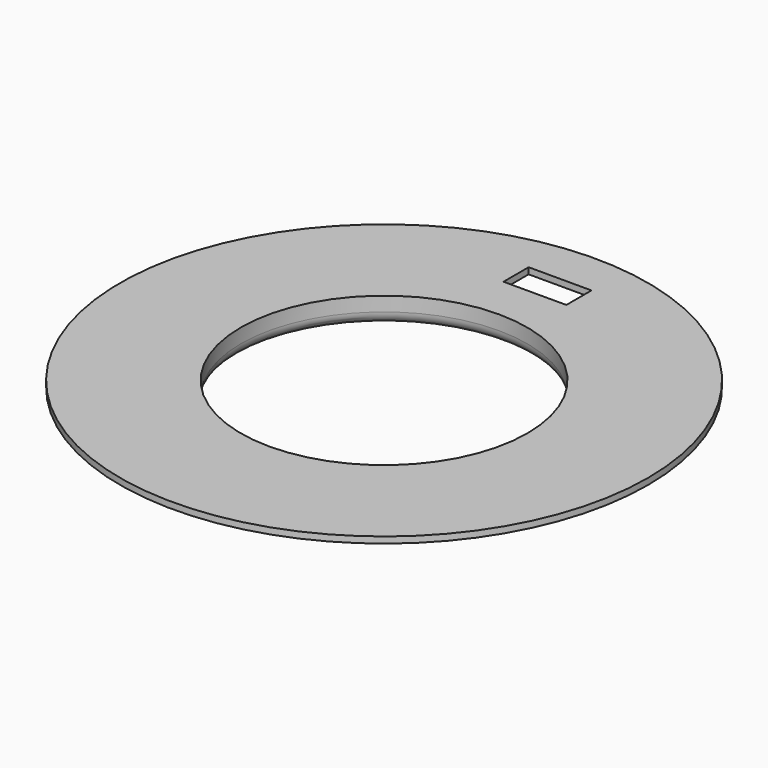
from build123d import *

# Parameters (mm, degrees)
F3_DEPTH = 25


# Not quite as in the source:
# - a fillet or chamfer that OpenCascade refuses, or shapes differently, is made with other operations: its cross-section is extruded or revolved along the edge and cut away or added


with BuildPart() as f1:
    # F0 (on Front) → F1 (revolve)
    with BuildSketch(Plane.XZ):
        Polygon((22.8, -3), (23.8, -3), (23.8, 0), (42, 0), (42, 1), (22.8, 1), align=None)
    revolve(axis=Axis((0, 0, 4.016155377), (0, 0, 1)))

    # F2 (on Top) → F3 (cut)
    with BuildSketch(Plane.XY):
        Polygon((-5, 30), (0, 30), (5, 30), (5, 35), (-5, 35), align=None)
    extrude(amount=F3_DEPTH, mode=Mode.SUBTRACT)

    # F4: fillet of radius 2 on 1 edges, made by hand

    # F4_s1 → F4_t2 (revolve, cut)
    with BuildSketch(Plane.XZ):
        with BuildLine():
            ThreePointArc((23.8, -3), (23.0679491924, -2.2679491924), (22.8, -1.2679491924))
            Line((22.8, -1.2679491924), (22.8, -3))
            Line((22.8, -3), (23.8, -3))
        make_face()
    revolve(axis=Axis((0, 0, -3), (0, 0, 1)), mode=Mode.SUBTRACT)


solid = f1.part
